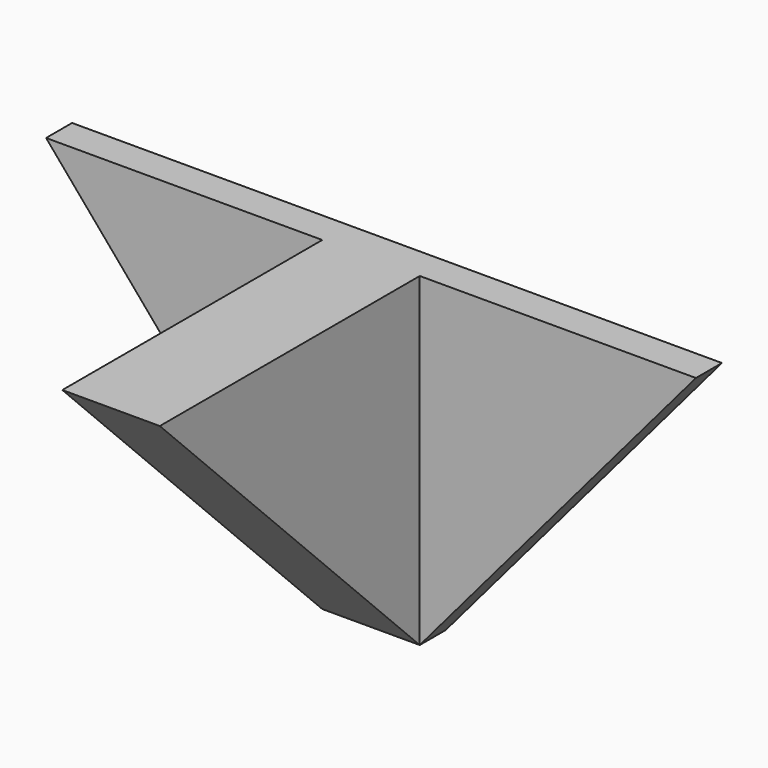
from build123d import *

# Parameters (mm, degrees)
F1_DEPTH = 10
F2_W     = 30
F2_H     = 100
F3_DEPTH = 100
F4_SIZE  = 99.99999


# Not quite as in the source:
# - a fillet or chamfer is up to 0.001 mm smaller than in the source, because OpenCascade refuses the exact size


with BuildPart() as f1:
    # F0 (on Front) → F1 (new body)
    with BuildSketch(Plane.XZ):
        Polygon((0, -100), (0, 0), (-100, 0), (-15, -100), align=None)
        Polygon((100, 0), (0, 0), (0, -100), (15, -100), align=None)
    extrude(amount=F1_DEPTH)

    # F2 (on face) → F3 (join)
    with BuildSketch(Plane.XZ.offset(10)):
        with Locations((0, -50)):
            Rectangle(F2_W, F2_H)
    extrude(amount=F3_DEPTH)

    # F4 (size 100 in the source; OpenCascade refuses exactly that, so slightly less here)
    f4_edges = [f1.edges().sort_by_distance(p)[0] for p in [
        (0, -110, -100),
    ]]
    chamfer(f4_edges, length=F4_SIZE)


solid = f1.part
